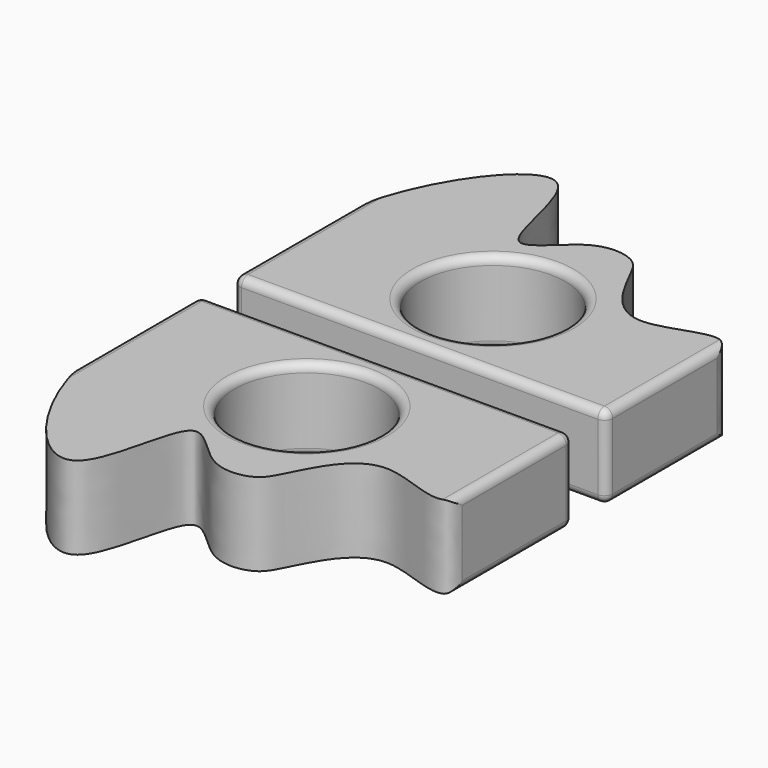
from build123d import *

# Parameters (mm, degrees)
F0_R         = 17.4427068078
F1_DEPTH     = 20
F2_T1_DEPTH  = 36.464721171
F2_T3_DEPTH  = 46.464721171
F2_T5_DEPTH  = 16
F2_T7_DEPTH  = 85.9132043123
F2_S11_W     = 2
F2_S11_H     = 2
F2_T12_DEPTH = 2
F2_S17_W     = 2
F2_S17_H     = 2
F2_T18_DEPTH = 2
F2_S23_W     = 2
F2_S23_H     = 2
F2_T24_DEPTH = 2
F2_S29_W     = 2
F2_S29_H     = 2
F2_T30_DEPTH = 2


# Not quite as in the source:
# - a fillet or chamfer that OpenCascade refuses, or shapes differently, is made with other operations: its cross-section is extruded or revolved along the edge and cut away or added


with BuildPart() as f1:
    # F0 (on Top) → F1 (new body)
    with BuildSketch(Plane.XY):
        with BuildLine():
            Line((-44.193431735, 33.464721171), (-44.193431735, 0))
            add(Edge.make_bspline(
                [(-44.193431735, 0), (-41.5374976489, -19.1170855808), (-15.8967697517, -53.4445438189), (-13.8709136066, -0.8359905473), (-0.6333739829, -20.4119289474), (10.1468025815, -19.2910154929), (13.9700006637, -14.7607486575), (23.3393930952, 8.7972644669), (45.1072581689, -8.0366569396), (45.7197725773, 0)],
                knots=[0, 0, 0, 0, 0.2201917148, 0.3911048075, 0.5128109298, 0.6182617293, 0.7019727801, 0.8530823003, 1, 1, 1, 1], degree=3))
            Line((45.7197725773, 0), (45.7197725773, 33.464721171))
            Line((45.7197725773, 33.464721171), (-44.193431735, 33.464721171))
        make_face()
        with Locations((0, 10.3995623067)):
            Circle(F0_R, mode=Mode.SUBTRACT)
    extrude(amount=F1_DEPTH)

    # F2: fillet of radius 2 on 10 edges, made by hand

    # F2_s2 → F2_t1 (cut)
    with BuildSketch(Plane.XZ.offset(-31.464721171)):
        with BuildLine():
            ThreePointArc((45.7197725773, 18), (45.1339861397, 19.4142135624), (43.7197725773, 20))
            Line((43.7197725773, 20), (45.7197725773, 20))
            Line((45.7197725773, 20), (45.7197725773, 18))
        make_face()
        with BuildLine():
            ThreePointArc((45.7197725773, 2), (45.1339861397, 0.5857864376), (43.7197725773, 0))
            Line((43.7197725773, 0), (45.7197725773, 0))
            Line((45.7197725773, 0), (45.7197725773, 2))
        make_face()
    extrude(amount=F2_T1_DEPTH, mode=Mode.SUBTRACT)

    # F2_s4 → F2_t3 (cut)
    with BuildSketch(Plane.XZ.offset(-31.464721171)):
        with BuildLine():
            ThreePointArc((-44.193431735, 18), (-43.6076452974, 19.4142135624), (-42.193431735, 20))
            Line((-42.193431735, 20), (-44.193431735, 20))
            Line((-44.193431735, 20), (-44.193431735, 18))
        make_face()
        with BuildLine():
            ThreePointArc((-44.193431735, 2), (-43.6076452974, 0.5857864376), (-42.193431735, 0))
            Line((-42.193431735, 0), (-44.193431735, 0))
            Line((-44.193431735, 0), (-44.193431735, 2))
        make_face()
    extrude(amount=F2_T3_DEPTH, mode=Mode.SUBTRACT)

    # F2_s6 → F2_t5 (cut)
    with BuildSketch(Plane.XY.offset(2)):
        with BuildLine():
            ThreePointArc((-42.193431735, 33.464721171), (-43.6076452974, 32.8789347334), (-44.193431735, 31.464721171))
            Line((-44.193431735, 31.464721171), (-44.193431735, 33.464721171))
            Line((-44.193431735, 33.464721171), (-42.193431735, 33.464721171))
        make_face()
        with BuildLine():
            ThreePointArc((43.7197725773, 33.464721171), (45.1339861397, 32.8789347334), (45.7197725773, 31.464721171))
            Line((45.7197725773, 31.464721171), (45.7197725773, 33.464721171))
            Line((45.7197725773, 33.464721171), (43.7197725773, 33.464721171))
        make_face()
    extrude(amount=F2_T5_DEPTH, mode=Mode.SUBTRACT)

    # F2_s8 → F2_t7 (cut)
    with BuildSketch(Plane.YZ.offset(-42.193431735)):
        with BuildLine():
            ThreePointArc((33.464721171, 2), (32.8789347334, 0.5857864376), (31.464721171, 0))
            Line((31.464721171, 0), (33.464721171, 0))
            Line((33.464721171, 0), (33.464721171, 2))
        make_face()
        with BuildLine():
            ThreePointArc((33.464721171, 18), (32.8789347334, 19.4142135624), (31.464721171, 20))
            Line((31.464721171, 20), (33.464721171, 20))
            Line((33.464721171, 20), (33.464721171, 18))
        make_face()
    extrude(amount=F2_T7_DEPTH, mode=Mode.SUBTRACT)


with BuildPart() as f2_tool10:
    # F2_s11 → F2_t12 (new body)
    with BuildSketch(Plane.XZ.offset(-31.464721171)):
        with Locations((44.7197725773, 19)):
            Rectangle(F2_S11_W, F2_S11_H)
    extrude(amount=-F2_T12_DEPTH)

    # F2_s13 → F2_t14 (revolve, cut)
    with BuildSketch(Plane(origin=(43.7197725773, 31.464721171, 18), x_dir=(-0.7071067812, 0, -0.7071067812), z_dir=(0.7071067812, 0, -0.7071067812))):
        with BuildLine():
            ThreePointArc((0, -2), (2, 0), (0, 2))
            Line((0, 2), (0, -2))
        make_face()
    revolve(axis=Axis((43.7197725773, 31.464721171, 18), (0, 1, 0)), mode=Mode.SUBTRACT)


with BuildPart() as f1_1:
    add(f1.part)

    # F2_t9: cut F2_tool10
    add(f2_tool10.part, mode=Mode.SUBTRACT)


with BuildPart() as f2_tool16:
    # F2_s17 → F2_t18 (new body)
    with BuildSketch(Plane.XZ.offset(-31.464721171)):
        with Locations((44.7197725773, 1)):
            Rectangle(F2_S17_W, F2_S17_H)
    extrude(amount=-F2_T18_DEPTH)

    # F2_s19 → F2_t20 (revolve, cut)
    with BuildSketch(Plane(origin=(43.7197725773, 31.464721171, 2), x_dir=(-0.7071067812, 0, 0.7071067812), z_dir=(-0.7071067812, 0, -0.7071067812))):
        with BuildLine():
            ThreePointArc((0, -2), (2, 0), (0, 2))
            Line((0, 2), (0, -2))
        make_face()
    revolve(axis=Axis((43.7197725773, 31.464721171, 2), (0, 1, 0)), mode=Mode.SUBTRACT)


with BuildPart() as f1_2:
    add(f1_1.part)

    # F2_t15: cut F2_tool16
    add(f2_tool16.part, mode=Mode.SUBTRACT)


with BuildPart() as f2_tool22:
    # F2_s23 → F2_t24 (new body)
    with BuildSketch(Plane.XZ.offset(-31.464721171)):
        with Locations((-43.193431735, 19)):
            Rectangle(F2_S23_W, F2_S23_H)
    extrude(amount=-F2_T24_DEPTH)

    # F2_s25 → F2_t26 (revolve, cut)
    with BuildSketch(Plane(origin=(-42.193431735, 31.464721171, 18), x_dir=(0.7071067812, 0, -0.7071067812), z_dir=(0.7071067812, 0, 0.7071067812))):
        with BuildLine():
            ThreePointArc((0, -2), (2, 0), (0, 2))
            Line((0, 2), (0, -2))
        make_face()
    revolve(axis=Axis((-42.193431735, 31.464721171, 18), (0, 1, 0)), mode=Mode.SUBTRACT)


with BuildPart() as f1_3:
    add(f1_2.part)

    # F2_t21: cut F2_tool22
    add(f2_tool22.part, mode=Mode.SUBTRACT)


with BuildPart() as f2_tool28:
    # F2_s29 → F2_t30 (new body)
    with BuildSketch(Plane.XZ.offset(-31.464721171)):
        with Locations((-43.193431735, 1)):
            Rectangle(F2_S29_W, F2_S29_H)
    extrude(amount=-F2_T30_DEPTH)

    # F2_s31 → F2_t32 (revolve, cut)
    with BuildSketch(Plane(origin=(-42.193431735, 31.464721171, 2), x_dir=(0.7071067812, 0, 0.7071067812), z_dir=(-0.7071067812, 0, 0.7071067812))):
        with BuildLine():
            ThreePointArc((0, -2), (2, 0), (0, 2))
            Line((0, 2), (0, -2))
        make_face()
    revolve(axis=Axis((-42.193431735, 31.464721171, 2), (0, 1, 0)), mode=Mode.SUBTRACT)


with BuildPart() as f1_4:
    add(f1_3.part)

    # F2_t27: cut F2_tool28
    add(f2_tool28.part, mode=Mode.SUBTRACT)

    # F2_s33 → F2_t34 (revolve, cut)
    with BuildSketch(Plane.XZ.offset(-10.3995623067)):
        with BuildLine():
            ThreePointArc((17.4427068078, 2), (18.0284932455, 0.5857864376), (19.4427068078, 0))
            Line((19.4427068078, 0), (17.4427068078, 0))
            Line((17.4427068078, 0), (17.4427068078, 2))
        make_face()
    revolve(axis=Axis((0, 10.3995623067, 0), (0, 0, 1)), mode=Mode.SUBTRACT)

    # F2_s35 → F2_t36 (revolve, cut)
    with BuildSketch(Plane.XZ.offset(-10.3995623067)):
        with BuildLine():
            ThreePointArc((17.4427068078, 18), (18.0284932455, 19.4142135624), (19.4427068078, 20))
            Line((19.4427068078, 20), (17.4427068078, 20))
            Line((17.4427068078, 20), (17.4427068078, 18))
        make_face()
    revolve(axis=Axis((0, 10.3995623067, 20), (0, 0, 1)), mode=Mode.SUBTRACT)


with BuildPart() as f3_1:
    # F3: instance of F1
    add(f1_4.part.mirror(Plane(origin=(0.7631704212, 33.464721171, 10), x_dir=(-1, 0, 0), z_dir=(0, 1, 0))))


with BuildPart() as f3_1_1:
    # F4: moved
    add(f3_1.part.moved(Location((0, 10, 0))))


solid = Compound([f1_4.part, f3_1_1.part])
